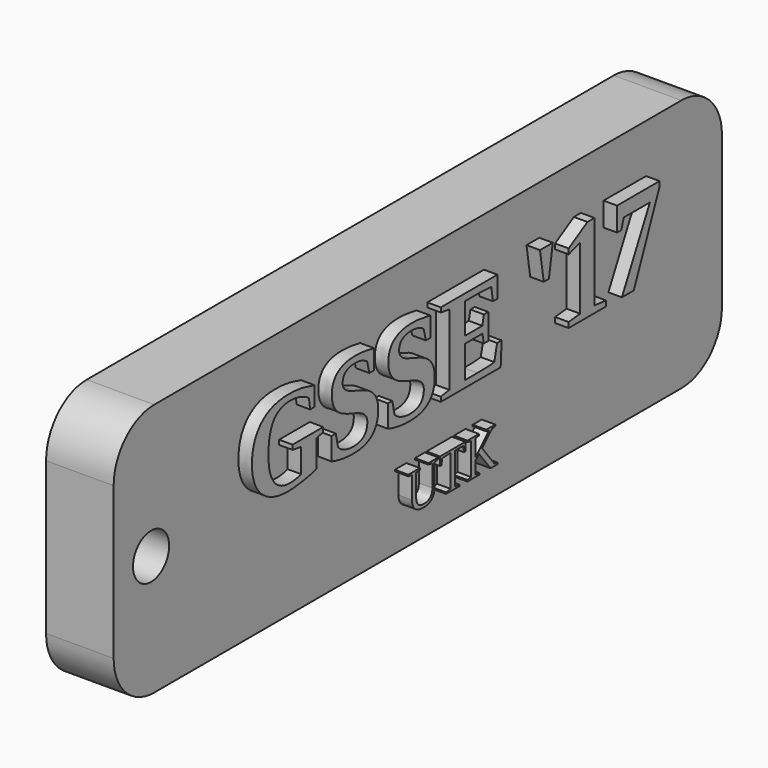
from build123d import *

# Parameters (mm, degrees)
F0_R           = 1.6988176655
F1_DEPTH       = 5.08
F2_TEXT_SIZE   = 9.54800764
F2_TEXT_SIZE_2 = 4.1413049783
F3_DEPTH       = 6.096


# Not quite as in the source:
# - Text() gives the source's letters only with a copy of the font that has no kerning and outlines rounded to 1/6400 em; it was checked with that copy


with BuildPart() as f1:
    # F0 (on Right) → F1 (new body)
    with BuildSketch(Plane.YZ):
        with BuildLine():
            Line((25.4359602935, 9.9115219028), (-24.0940397065, 9.9115219028))
            ThreePointArc((-24.0940397065, 9.9115219028), (-26.7881165428, 8.7955987392), (-27.9040397065, 6.1015219028))
            Line((-27.9040397065, 6.1015219028), (-27.9040397065, -5.3284780972))
            ThreePointArc((-27.9040397065, -5.3284780972), (-26.7881165428, -8.0225549335), (-24.0940397065, -9.1384780972))
            Line((-24.0940397065, -9.1384780972), (25.4359602935, -9.1384780972))
            ThreePointArc((25.4359602935, -9.1384780972), (28.1300371298, -8.0225549335), (29.2459602935, -5.3284780972))
            Line((29.2459602935, -5.3284780972), (29.2459602935, 6.1015219028))
            ThreePointArc((29.2459602935, 6.1015219028), (28.1300371298, 8.7955987392), (25.4359602935, 9.9115219028))
        make_face()
        with Locations((-24.3887100369, 0)):
            Circle(F0_R, mode=Mode.SUBTRACT)
    extrude(amount=F1_DEPTH)

    # F2 (on Right) → F3 (join)
    with BuildSketch(Plane.YZ):
        with Locations((-16.6480429471, 0)):
            Text("GSSE '17", F2_TEXT_SIZE, font='Tinos', font_style=FontStyle.BOLD, text_align=(TextAlign.LEFT, TextAlign.BOTTOM))
        with Locations((-1.5736961068, -6.2947827391)):
            Text('UTK', F2_TEXT_SIZE_2, font='Tinos', text_align=(TextAlign.LEFT, TextAlign.BOTTOM))
    extrude(amount=F3_DEPTH)


solid = f1.part
